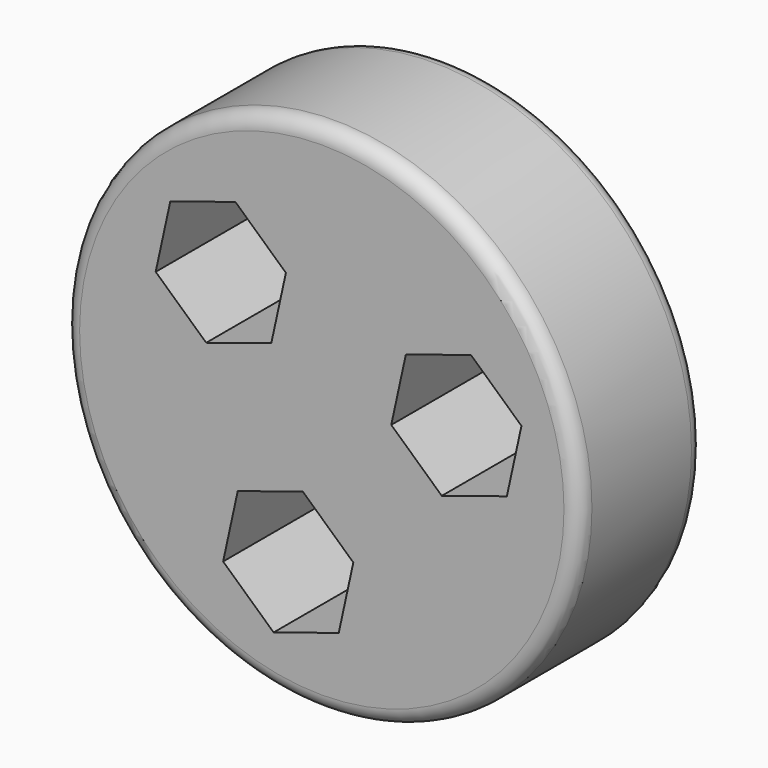
from build123d import *

# Parameters (mm, degrees)
F0_R            = 42.0966561171
F1_DEPTH        = 25.4
F3_DEPTH        = 25.401
F3_COPIES_COUNT = 3
F4_R            = 2.54
F5_R            = 2.54


# Not quite as in the source:
# - a pattern or mirror of a feature is missing from the dataset's text; its kind, count and spacing are read off the source's solid


with BuildPart() as f1:
    # F0 (on Front) → F1 (new body)
    with BuildSketch(Plane.XZ):
        Circle(F0_R)
    extrude(amount=F1_DEPTH)

    # F2 (on face) → F3 (cut, through all)
    with BuildSketch(Plane.XZ.offset(25.4)):
        Polygon((-18.881084953, 4.9543602206), (-8.2484530285, 8.3401026204), (-5.8642759952, 19.241103176), (-14.1127308863, 26.7563613318), (-24.7453628108, 23.3706189319), (-27.1295398441, 12.4696183764), align=None)
    f3 = extrude(amount=-F3_DEPTH, mode=Mode.SUBTRACT)

    # F3_copies: F3 ×3 about axis
    f3_copies_axis = Axis((0, 0, 0), (0, 1, 0))
    for i in range(1, F3_COPIES_COUNT):
        add(f3.rotate(f3_copies_axis, i * 360 / F3_COPIES_COUNT), mode=Mode.SUBTRACT)

    # F4
    f4_edges = [f1.edges().sort_by_distance(p)[0] for p in [
        (-42.096656, -25.4, 0),
    ]]
    fillet(f4_edges, radius=F4_R)

    # F5
    f5_edges = [f1.edges().sort_by_distance(p)[0] for p in [
        (-42.096656, 0, 0),
    ]]
    fillet(f5_edges, radius=F5_R)


solid = f1.part
